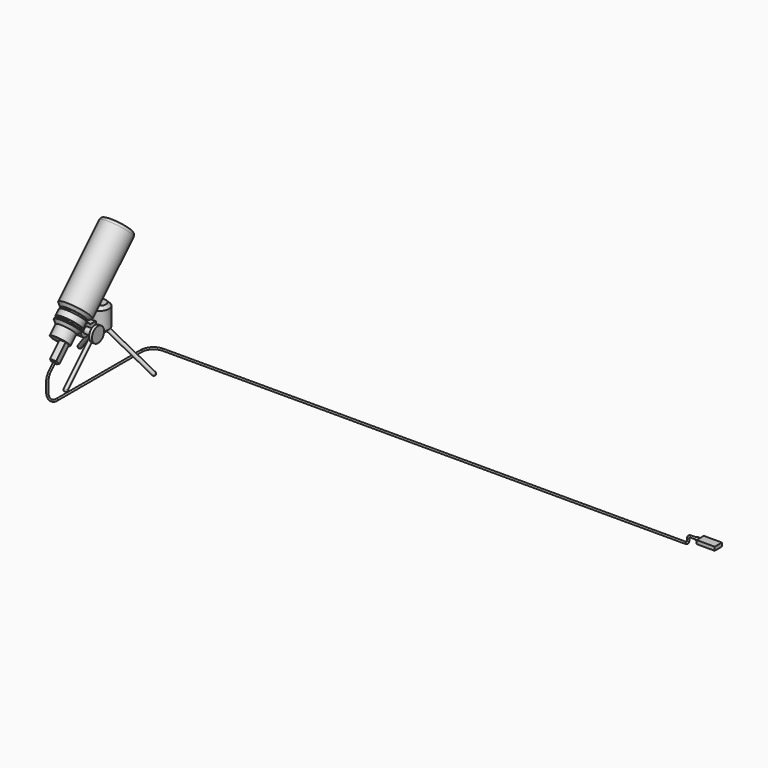
from build123d import *

# Parameters (mm, degrees)
F0_R      = 15
F1_DEPTH  = 40
F2_SIZE   = 5
F12_W     = 10
F12_H     = 10
F13_DEPTH = 30
F15_DEPTH = 5
F16_R     = 20
F17_DEPTH = 10
F20_R     = 5
F21_SIZE  = 4.99999
F22_R     = 5
F23_DEPTH = 15
F24_R     = 12.5
F25_DEPTH = 5
F26_W     = 10
F26_H     = 10
F27_DEPTH = 30
F28_SIZE  = 2
F30_R     = 1.5
F32_R     = 1.5
F36_R     = 1.5
F40_W     = 15
F40_H     = 6
F41_DEPTH = 30
F42_R     = 2.5
F43_DEPTH = 6


# Not quite as in the source:
# - a fillet or chamfer is up to 0.001 mm smaller than in the source, because OpenCascade refuses the exact size


with BuildPart() as f1:
    # F0 (on Top) → F1 (new body)
    with BuildSketch(Plane.XY):
        Circle(F0_R)
    extrude(amount=F1_DEPTH)

    # F2
    f2_edges = [f1.edges().sort_by_distance(p)[0] for p in [
        (-15, 0, 0),
        (-15, 0, 40),
    ]]
    chamfer(f2_edges, length=F2_SIZE)

    # F3 (on Right) → F4 (revolve)
    with BuildSketch(Plane.YZ):
        with BuildLine():
            Line((-2.1213203436, 14.1213203436), (-72.8319984622, -56.5893577751))
            ThreePointArc((-72.8319984622, -56.5893577751), (-73.7106781187, -58.7106781187), (-72.8319984622, -60.8319984622))
            Line((-72.8319984622, -60.8319984622), (0, 12))
            Line((0, 12), (-2.1213203436, 14.1213203436))
        make_face()
    revolve(axis=Axis((0, -36.4159992311, -24.4159992311), (0, 0.7071067812, 0.7071067812)))

    # F7 (on line) → F8 (revolve)
    with BuildSketch(Plane(origin=(0, 0, 0), x_dir=(0.8660254038, 0.5, 0), z_dir=(0.5, -0.8660254038, 0))):
        with BuildLine():
            Line((2.0230960578, 14.2195446293), (0, 12))
            Line((0, 12), (72.7337741765, -60.7337741765))
            ThreePointArc((72.7337741765, -60.7337741765), (73.6124538329, -58.6124538329), (72.7337741765, -56.4911334894))
            Line((72.7337741765, -56.4911334894), (2.0230960578, 14.2195446293))
        make_face()
    revolve(axis=Axis((31.494648075, 18.1834435441, -24.3668870882), (0.6123724357, 0.3535533906, -0.7071067812)))

    # F10 (on face) → F11 (revolve)
    with BuildSketch(Plane(origin=(0, 0, 0), x_dir=(0.8660254038, -0.5, 0), z_dir=(-0.5, -0.8660254038, 0))):
        with BuildLine():
            Line((-72.8869811403, -60.8869811403), (0, 12))
            Line((0, 12), (-2.1763030217, 14.0663376655))
            Line((-2.1763030217, 14.0663376655), (-72.8869811403, -56.6443404532))
            ThreePointArc((-72.8869811403, -56.6443404532), (-73.7656607968, -58.7656607968), (-72.8869811403, -60.8869811403))
        make_face()
    revolve(axis=Axis((-31.5609886363, 18.2217452851, -24.4434905702), (-0.6123724357, 0.3535533906, -0.7071067812)))

    # F12 (on Front) → F13 (join)
    with BuildSketch(Plane.XZ):
        with Locations((0, 15)):
            Rectangle(F12_W, F12_H)
    extrude(amount=F13_DEPTH)

    # F14 (on Right) → F15 (join, symmetric)
    with BuildSketch(Plane.YZ):
        with BuildLine():
            ThreePointArc((-44.6592582629, 17.588190451), (-36.3052619222, 5.0855513863), (-25, 15))
            ThreePointArc((-25, 15), (-28.9123857099, 22.9335334029), (-37.588190451, 24.6592582629))
            Line((-37.588190451, 24.6592582629), (-31.4644660941, 18.5355339059))
            Line((-31.4644660941, 18.5355339059), (-35, 15))
            Line((-35, 15), (-38.5355339059, 11.4644660941))
            Line((-38.5355339059, 11.4644660941), (-44.6592582629, 17.588190451))
        make_face()
        with BuildLine():
            Line((-31.4644660941, 18.5355339059), (-37.588190451, 24.6592582629))
            ThreePointArc((-37.588190451, 24.6592582629), (-42.0710678119, 22.0710678119), (-44.6592582629, 17.588190451))
            Line((-44.6592582629, 17.588190451), (-38.5355339059, 11.4644660941))
            Line((-38.5355339059, 11.4644660941), (-35, 15))
            Line((-35, 15), (-31.4644660941, 18.5355339059))
        make_face()
        with BuildLine():
            ThreePointArc((-44.6592582629, 17.588190451), (-42.0710678119, 22.0710678119), (-37.588190451, 24.6592582629))
            Line((-37.588190451, 24.6592582629), (-45.6066017178, 32.6776695297))
            Line((-45.6066017178, 32.6776695297), (-52.6776695297, 25.6066017178))
            Line((-52.6776695297, 25.6066017178), (-44.6592582629, 17.588190451))
        make_face()
    extrude(amount=F15_DEPTH, both=True)

    # F16 (on face) → F17 (join)
    with BuildSketch(Plane(origin=(0, -6.4644660941, -6.4644660941), x_dir=(1, 0, 0), z_dir=(0, 0.7071067812, 0.7071067812))):
        with Locations((0, -70.3553390593)):
            Circle(F16_R)
    extrude(amount=-F17_DEPTH)

    # F18 (on Right) → F19 (revolve)
    with BuildSketch(Plane.YZ):
        Polygon((-89.4472221514, 24.1923881554), (-82.3761543395, 17.1213203436), (37.8319984622, 137.3294731453), (20.1543289326, 155.0071426749), (-71.7695526217, 63.0832611207), (-66.1126983722, 57.4264068712), (-77.4264068712, 46.1126983722), (-79.5477272148, 48.2340187158), (-84.4974746831, 43.2842712475), (-80.9619407771, 39.7487373415), (-92.9827560573, 27.7279220614), align=None)
    revolve(axis=Axis((0, -22.2720779386, 77.2253967444), (0, 0.7071067812, 0.7071067812)))

    # F20
    f20_edges = [f1.edges().sort_by_distance(p)[0] for p in [
        (0, 55.509668, 119.651804),
    ]]
    fillet(f20_edges, radius=F20_R)

    # F21 (size 5 in the source; OpenCascade refuses exactly that, so slightly less here)
    f21_edges = [f1.edges().sort_by_distance(p)[0] for p in [
        (0, -36.414214, 27.727922),
        (0, -56.213203, 15),
    ]]
    chamfer(f21_edges, length=F21_SIZE)

    # F22 (on face) → F23 (join)
    with BuildSketch(Plane.YZ.offset(5)):
        with Locations((-35, 15)):
            Circle(F22_R)
    extrude(amount=F23_DEPTH)

    # F24 (on face) → F25 (join)
    with BuildSketch(Plane.YZ.offset(20)):
        with Locations((-35, 15)):
            Circle(F24_R)
    extrude(amount=F25_DEPTH)

    # F26 (on face) → F27 (join)
    with BuildSketch(Plane(origin=(0, -32.627416998, -32.627416998), x_dir=(1, 0, 0), z_dir=(0, -0.7071067812, -0.7071067812))):
        with Locations((7, 70.3553390593)):
            Rectangle(F26_W, F26_H)
    extrude(amount=F27_DEPTH)

    # F28
    f28_edges = [f1.edges().sort_by_distance(p)[0] for p in [
        (2, -103.589358, -4.091883),
        (7, -100.053824, -7.627417),
        (12, -103.589358, -4.091883),
        (7, -107.124892, -0.556349),
    ]]
    chamfer(f28_edges, length=F28_SIZE)

    # F31: sweep along a path in F29
    with BuildLine(Plane.YZ) as f31_path:
        Line((-103.5893577751, -4.091883092), (-111.8736290226, -12.3761543395))
        ThreePointArc((-111.8736290226, -12.3761543395), (-116.2090840491, -18.8646213159), (-117.7314933988, -26.5182899632))
        Line((-117.7314933988, -26.5182899632), (-117.7314933988, -40.2340187158))
        ThreePointArc((-117.7314933988, -40.2340187158), (-111.8736290226, -54.3761543395), (-97.7314933988, -60.2340187158))
        Line((-97.7314933988, -60.2340187158), (72.2685066012, -60.2340187158))
    # F30 (on face) → F31 (sweep)
    with BuildSketch(Plane(origin=(0, -53.8406204336, -53.8406204336), x_dir=(1, 0, 0), z_dir=(0, -0.7071067812, -0.7071067812))):
        with Locations((7, 70.3553390593)):
            Circle(F30_R)
    sweep(path=f31_path.line)

    # F35: sweep along a path in F34
    with BuildLine(Plane.XY.offset(-60.2340187158)) as f35_path:
        Line((877, 97.2685066012), (27, 97.2685066012))
        ThreePointArc((27, 97.2685066012), (12.8578643763, 91.4106422249), (7, 77.2685066012))
        Line((7, 77.2685066012), (7, 72.2685066012))
    # F32 (on face) → F35 (sweep)
    with BuildSketch(Plane(origin=(0, 72.2685066012, 0), x_dir=(-1, 0, 0), z_dir=(0, 1, 0))):
        with Locations((-7, -60.2340187158)):
            Circle(F32_R)
    sweep(path=f35_path.line)

    # F39: sweep along a path in F38
    with BuildLine(Plane(origin=(0, 97.2685066012, 0), x_dir=(-1, 0, 0), z_dir=(0, 1, 0))) as f39_path:
        Line((-877, -60.2340187158), (-893, -60.2340187158))
        ThreePointArc((-893, -60.2340187158), (-895.8284271247, -59.0624458405), (-897, -56.2340187158))
        Line((-897, -56.2340187158), (-897, -52.2340187158))
        ThreePointArc((-897, -52.2340187158), (-898.1715728753, -49.405591591), (-901, -48.2340187158))
        Line((-901, -48.2340187158), (-917, -48.2340187158))
    # F36 (on face) → F39 (sweep)
    with BuildSketch(Plane.YZ.offset(877)):
        with Locations((97.2685066012, -60.2340187158)):
            Circle(F36_R)
    sweep(path=f39_path.line)

    # F40 (on face) → F41 (join)
    with BuildSketch(Plane.YZ.offset(917)):
        with Locations((97.2685066012, -48.2340187158)):
            Rectangle(F40_W, F40_H)
    extrude(amount=F41_DEPTH)

    # F42 (on face) → F43 (join)
    with BuildSketch(Plane(origin=(917, 0, 0), x_dir=(0, -1, 0), z_dir=(-1, 0, 0))):
        with Locations((-97.2685066012, -48.2340187158)):
            Circle(F42_R)
    extrude(amount=F43_DEPTH)


solid = f1.part
